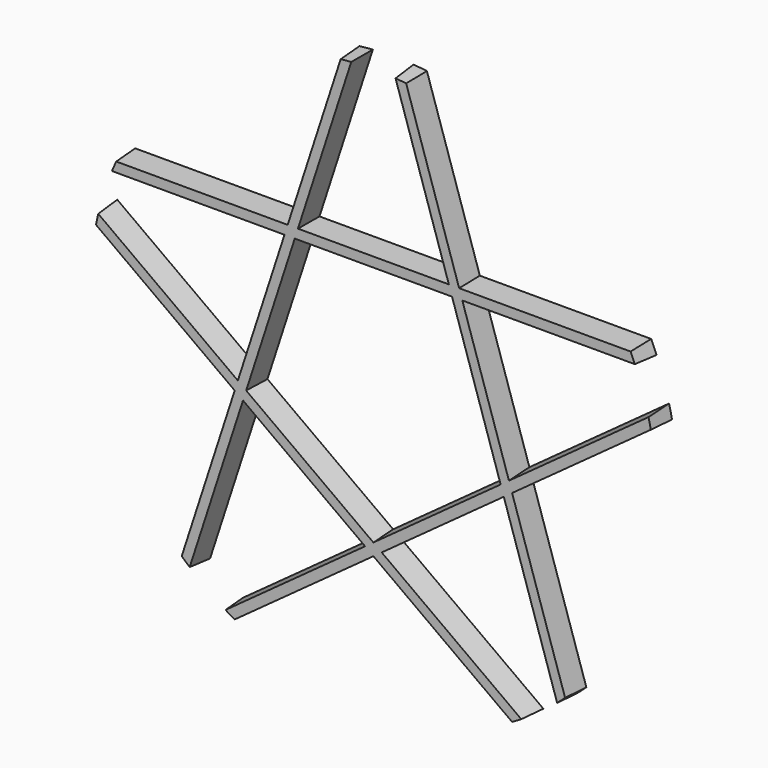
from build123d import *

# Parameters (mm, degrees)
F1_DEPTH               = 12.7
DRAFT_F1_DRAFTED_ANGLE = 3


# Not quite as in the source:
# - an extrude with a draft is written as a straight extrude whose walls are then drafted


with BuildPart() as f1:
    # F0 (on Front) → F1 (new body)
    with BuildSketch(Plane.XZ):
        with BuildLine():
            Line((72.0545034438, -23.4119273712), (143.2753959432, 28.3330799122))
            ThreePointArc((143.2753959432, 28.3330799122), (142.5637423713, 31.7203698132), (141.7720188707, 35.0898441905))
            Line((141.7720188707, 35.0898441905), (69.9912633727, -17.0619273712))
            Line((69.9912633727, -17.0619273712), (72.0545034438, -23.4119273712))
        make_face()
        with BuildLine():
            ThreePointArc((94.0706796729, -111.71978216), (96.6917247866, -109.4591835242), (99.2584636695, -107.1371079037))
            Line((99.2584636695, -107.1371079037), (72.0545034438, -23.4119273712))
            Line((72.0545034438, -23.4119273712), (66.6528708108, -27.3364431997))
            Line((66.6528708108, -27.3364431997), (94.0706796729, -111.71978216))
        make_face()
        Polygon((66.6528708108, -27.3364431997), (72.0545034438, -23.4119273712), (69.9912633727, -17.0619273712), (64.5896307397, -20.9864431997), align=None)
        with BuildLine():
            Line((46.5953722418, 54.9432215999), (135.3212655137, 54.9432215999))
            ThreePointArc((135.3212655137, 54.9432215999), (133.9812559336, 58.1345470307), (132.5659967183, 61.2932215999))
            Line((132.5659967183, 61.2932215999), (44.5321321708, 61.2932215999))
            Line((44.5321321708, 61.2932215999), (46.5953722418, 54.9432215999))
        make_face()
        Polygon((64.5896307397, -20.9864431997), (69.9912633727, -17.0619273712), (46.5953722418, 54.9432215999), (39.9185871179, 54.9432215999), align=None)
        Polygon((5.401632633, -71.8380726288), (66.6528708108, -27.3364431997), (64.5896307397, -20.9864431997), (0, -67.9135568003), align=None)
        with BuildLine():
            ThreePointArc((71.2208924994, -127.5075957407), (74.2224835846, -125.7840428295), (77.1823881311, -123.9898441905))
            Line((77.1823881311, -123.9898441905), (5.401632633, -71.8380726288))
            Line((5.401632633, -71.8380726288), (0, -75.7625884574))
            Line((0, -75.7625884574), (71.2208924994, -127.5075957407))
        make_face()
        Polygon((39.9185871179, 54.9432215999), (46.5953722418, 54.9432215999), (44.5321321708, 61.2932215999), (37.8553470468, 61.2932215999), align=None)
        Polygon((0, -75.7625884574), (5.401632633, -71.8380726288), (0, -67.9135568003), (-5.401632633, -71.8380726288), align=None)
        with BuildLine():
            Line((44.5321321708, 61.2932215999), (17.3281719451, 145.0184021324))
            ThreePointArc((17.3281719451, 145.0184021324), (13.8867547642, 145.3883095098), (10.4375381847, 145.6765605602))
            Line((10.4375381847, 145.6765605602), (37.8553470468, 61.2932215999))
            Line((37.8553470468, 61.2932215999), (44.5321321708, 61.2932215999))
        make_face()
        Polygon((-39.9185871179, 54.9432215999), (39.9185871179, 54.9432215999), (37.8553470468, 61.2932215999), (-37.8553470468, 61.2932215999), align=None)
        Polygon((-5.401632633, -71.8380726288), (0, -67.9135568003), (-64.5896307397, -20.9864431997), (-66.6528708108, -27.3364431997), align=None)
        with BuildLine():
            Line((-71.2208924994, -127.5075957407), (0, -75.7625884574))
            Line((0, -75.7625884574), (-5.401632633, -71.8380726288))
            Line((-5.401632633, -71.8380726288), (-77.1823881311, -123.9898441905))
            ThreePointArc((-77.1823881311, -123.9898441905), (-74.2224835846, -125.7840428295), (-71.2208924994, -127.5075957407))
        make_face()
        Polygon((-46.5953722418, 54.9432215999), (-39.9185871179, 54.9432215999), (-37.8553470468, 61.2932215999), (-44.5321321708, 61.2932215999), align=None)
        Polygon((-64.5896307397, -20.9864431997), (-39.9185871179, 54.9432215999), (-46.5953722418, 54.9432215999), (-69.9912633727, -17.0619273712), align=None)
        Polygon((-66.6528708108, -27.3364431997), (-64.5896307397, -20.9864431997), (-69.9912633727, -17.0619273712), (-72.0545034438, -23.4119273712), align=None)
        with BuildLine():
            Line((-37.8553470468, 61.2932215999), (-10.4375381847, 145.6765605602))
            ThreePointArc((-10.4375381847, 145.6765605602), (-13.8867547642, 145.3883095098), (-17.3281719451, 145.0184021324))
            Line((-17.3281719451, 145.0184021324), (-44.5321321708, 61.2932215999))
            Line((-44.5321321708, 61.2932215999), (-37.8553470468, 61.2932215999))
        make_face()
        with BuildLine():
            Line((-135.3212655137, 54.9432215999), (-46.5953722418, 54.9432215999))
            Line((-46.5953722418, 54.9432215999), (-44.5321321708, 61.2932215999))
            Line((-44.5321321708, 61.2932215999), (-132.5659967183, 61.2932215999))
            ThreePointArc((-132.5659967183, 61.2932215999), (-133.9812559336, 58.1345470307), (-135.3212655137, 54.9432215999))
        make_face()
        with BuildLine():
            Line((-94.0706796729, -111.71978216), (-66.6528708108, -27.3364431997))
            Line((-66.6528708108, -27.3364431997), (-72.0545034438, -23.4119273712))
            Line((-72.0545034438, -23.4119273712), (-99.2584636695, -107.1371079037))
            ThreePointArc((-99.2584636695, -107.1371079037), (-96.6917247866, -109.4591835242), (-94.0706796729, -111.71978216))
        make_face()
        with BuildLine():
            Line((-72.0545034438, -23.4119273712), (-69.9912633727, -17.0619273712))
            Line((-69.9912633727, -17.0619273712), (-141.7720188707, 35.0898441905))
            ThreePointArc((-141.7720188707, 35.0898441905), (-142.5637423713, 31.7203698132), (-143.2753959432, 28.3330799122))
            Line((-143.2753959432, 28.3330799122), (-72.0545034438, -23.4119273712))
        make_face()
    extrude(amount=F1_DEPTH)

    # draft_F1_drafted
    draft_f1_drafted_walls = [f1.faces().sort_by_distance(p)[0] for p in [
        (-36.0272517219, -8.4666666667, -49.5872579143),
        (-41.2920103821, -8.4666666667, -97.9139584097),
        (-74.2224835846, -8.4666666667, -125.7840428295),
        (-35.6104462497, -8.4666666667, -101.6350920991),
        (35.6104462497, -8.4666666667, -101.6350920991),
        (74.2224835846, -8.4666666667, -125.7840428295),
        (41.2920103821, -8.4666666667, -97.9139584097),
        (36.0272517219, -8.4666666667, -49.5872579143),
        (80.3617752418, -8.4666666667, -69.5281126799),
        (96.6917247866, -8.4666666667, -109.4591835242),
        (85.6564835566, -8.4666666667, -65.2745176374),
        (107.6649496935, -8.4666666667, 2.4605762705),
        (142.5637423713, -8.4666666667, 31.7203698132),
        (105.8816411217, -8.4666666667, 9.0139584097),
        (58.2933178073, -8.4666666667, 18.9406471143),
        (90.9583188778, -8.4666666667, 54.9432215999),
        (133.9812559336, -8.4666666667, 58.1345470307),
        (88.5490644445, -8.4666666667, 61.2932215999),
        (30.9301520579, -8.4666666667, 103.1558118661),
        (13.8867547642, -8.4666666667, 145.3883095098),
        (24.1464426158, -8.4666666667, 103.48489108),
        (0, -8.4666666667, 61.2932215999),
        (-24.1464426158, -8.4666666667, 103.48489108),
        (-13.8867547642, -8.4666666667, 145.3883095098),
        (-30.9301520579, -8.4666666667, 103.1558118661),
        (-88.5490644445, -8.4666666667, 61.2932215999),
        (-133.9812559336, -8.4666666667, 58.1345470307),
        (-90.9583188778, -8.4666666667, 54.9432215999),
        (-58.2933178073, -8.4666666667, 18.9406471143),
        (-105.8816411217, -8.4666666667, 9.0139584097),
        (-142.5637423713, -8.4666666667, 31.7203698132),
        (-107.6649496935, -8.4666666667, 2.4605762705),
        (-85.6564835566, -8.4666666667, -65.2745176374),
        (-96.6917247866, -8.4666666667, -109.4591835242),
        (-80.3617752418, -8.4666666667, -69.5281126799),
        (-32.2948153698, -8.4666666667, -44.45),
        (-52.2541089288, -8.4666666667, 16.9783892001),
        (0, -8.4666666667, 54.9432215999),
        (52.2541089288, -8.4666666667, 16.9783892001),
        (32.2948153698, -8.4666666667, -44.45),
    ]]
    draft(draft_f1_drafted_walls, neutral_plane=Plane.XZ, angle=DRAFT_F1_DRAFTED_ANGLE)


solid = f1.part
